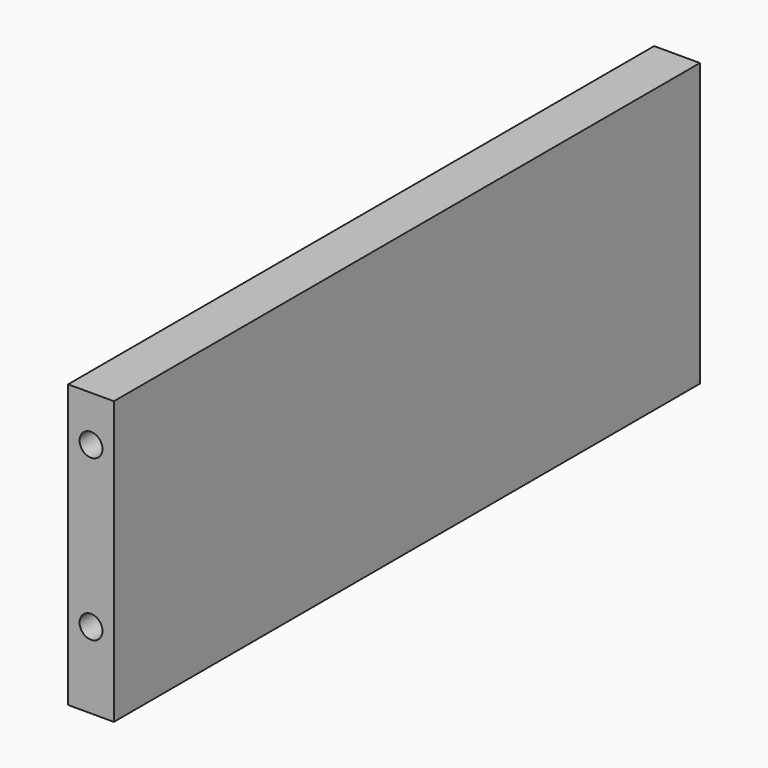
from build123d import *

# Parameters (mm, degrees)
F0_W     = 6
F0_H     = 96
F1_DEPTH = 37
F7_D     = 3
F7_DEPTH = 15
F7_TIP   = 0.9012909285
F9_D     = 3
F9_DEPTH = 15
F9_TIP   = 0.9012909285


# Not quite as in the source:
# - a feature of the source that left no trace in its solid (it failed there, or was rolled back) is left out


with BuildPart() as f1:
    # F0 (on Top) → F1 (new body)
    with BuildSketch(Plane.XY):
        with Locations((3, 48)):
            Rectangle(F0_W, F0_H)
    extrude(amount=F1_DEPTH)

    # F7
    with Locations(Plane.XZ):
        with Locations((3, 31), (3, 10)):
            Hole(F7_D / 2, depth=F7_DEPTH)
            with Locations((0, 0, -(F7_DEPTH + F7_TIP / 2))):  # 118° drill point
                Cone(0, F7_D / 2, F7_TIP, mode=Mode.SUBTRACT)

    # F9
    with Locations(Plane(origin=(0, 96, 0), x_dir=(-1, 0, 0), z_dir=(0, 1, 0))):
        with Locations((-3, 10), (-3, 31)):
            Hole(F9_D / 2, depth=F9_DEPTH)
            with Locations((0, 0, -(F9_DEPTH + F9_TIP / 2))):  # 118° drill point
                Cone(0, F9_D / 2, F9_TIP, mode=Mode.SUBTRACT)


solid = f1.part
